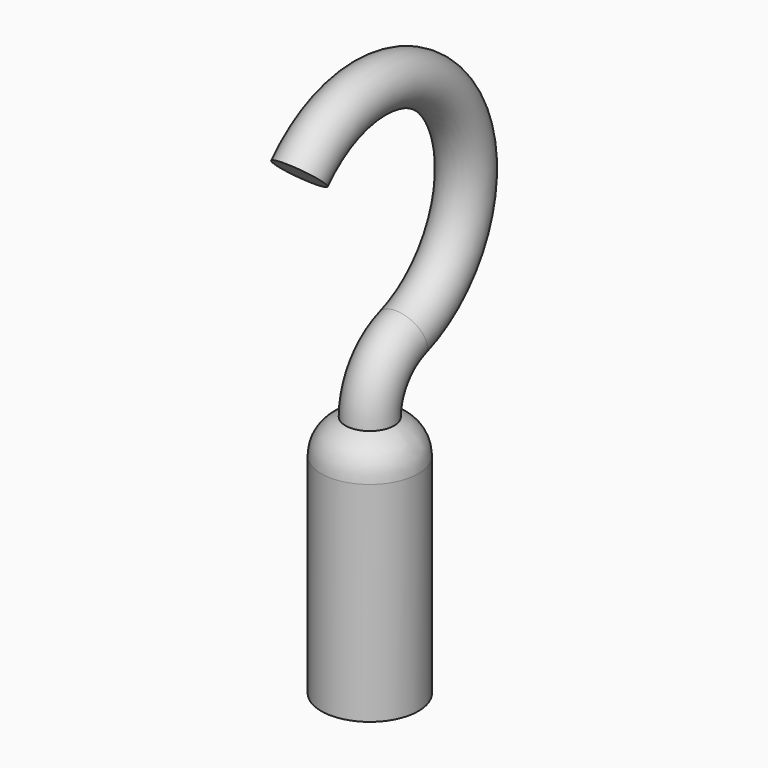
from build123d import *

# Parameters (mm, degrees)
F0_R     = 4
F3_R     = 2
F6_R     = 2
F7_DEPTH = 10


# Not quite as in the source:
# - a fillet or chamfer that OpenCascade refuses, or shapes differently, is made with other operations: its cross-section is extruded or revolved along the edge and cut away or added


with BuildPart() as f2:
    # F2: sweep along a path in F1
    with BuildLine(Plane.YZ) as f2_path:
        Line((0, 0), (0, 20.0361318752))
    # F0 (on Top) → F2 (sweep)
    with BuildSketch(Plane.XY):
        Circle(F0_R)
    sweep(path=f2_path.line)

    # F4: sweep along a path in F1
    with BuildLine(Plane.YZ) as f4_path:
        ThreePointArc((0, 20.0361318752), (0.9181759559, 22.9238147652), (3.3354849893, 24.7509372561))
        ThreePointArc((3.3354849893, 24.7509372561), (8.2388991441, 39.4795133809), (-7.2441254742, 40.5977144837))
    # F3 (on face) → F4 (sweep)
    with BuildSketch(Plane.XY.offset(20.0361318752)):
        Circle(F3_R)
    sweep(path=f4_path.line)

    # F5: fillet of radius 3 on 1 edges, made by hand

    # F5_s1 → F5_t2 (revolve, cut)
    with BuildSketch(Plane.XZ):
        with BuildLine():
            ThreePointArc((4, 17.2077047505), (3.4494897428, 18.939755558), (2, 20.0361318752))
            Line((2, 20.0361318752), (2.02, 20.0927004177))
            ThreePointArc((2.02, 20.0927004177), (3, 20.0961318752), (4, 20.0961318752))
            Line((4, 20.0961318752), (4.06, 20.0361318752))
            Line((4.06, 20.0361318752), (4.06, 17.2077047505))
            Line((4.06, 17.2077047505), (4, 17.2077047505))
        make_face()
    revolve(axis=Axis((0, 0, 20.0361318752), (0, 0, 1)), mode=Mode.SUBTRACT)

    # F6 (on face) → F7 (cut)
    with BuildSketch(Plane(origin=(0, 0, 0), x_dir=(1, 0, 0), z_dir=(0, 0, -1))):
        Circle(F6_R)
    extrude(amount=-F7_DEPTH, mode=Mode.SUBTRACT)


solid = f2.part
